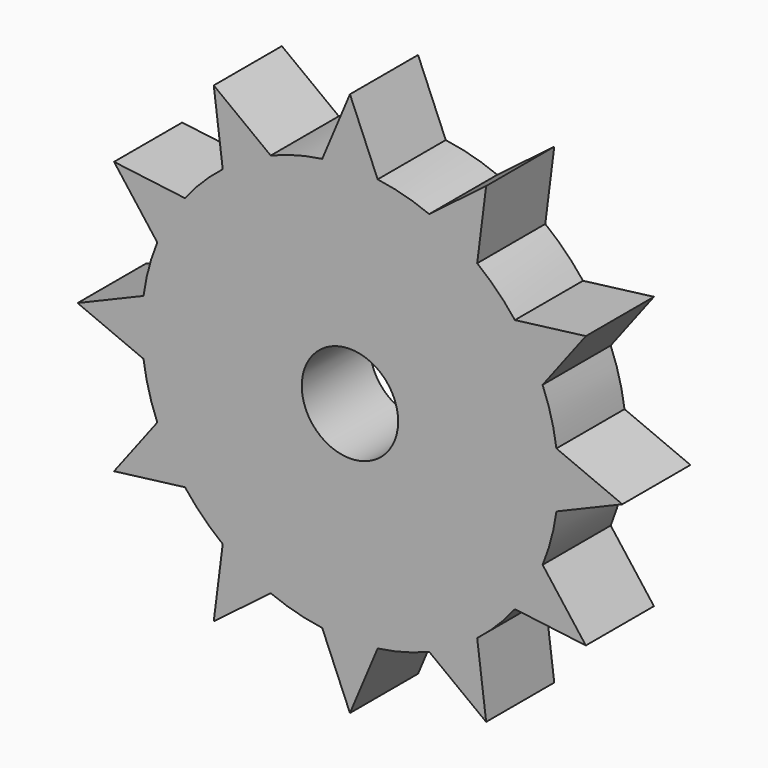
from build123d import *

# Parameters (mm, degrees)
F0_R            = 61.184507213
F1_DEPTH        = 25
F2_R            = 14.1604507034
F3_DEPTH        = 25
F5_DEPTH        = 25
F5_COPIES_COUNT = 12


# Not quite as in the source:
# - a pattern or mirror of a feature is missing from the dataset's text; its kind, count and spacing are read off the source's solid


with BuildPart() as f1:
    # F0 (on Front) → F1 (new body)
    with BuildSketch(Plane.XZ):
        Circle(F0_R)
    extrude(amount=F1_DEPTH)

    # F2 (on face) → F3 (cut)
    with BuildSketch(Plane.XZ.offset(25)):
        Circle(F2_R)
    extrude(amount=-F3_DEPTH, mode=Mode.SUBTRACT)

    # F4 (on Front) → F5 (join)
    with BuildSketch(Plane.XZ):
        with BuildLine():
            Line((0, 80), (-8.1378884566, 60.6408995181))
            ThreePointArc((-8.1378884566, 60.6408995181), (0, 61.184507213), (8.1378884566, 60.6408995181))
            Line((8.1378884566, 60.6408995181), (0, 80))
        make_face()
    f5 = extrude(amount=F5_DEPTH)

    # F5_copies: F5 ×12 about axis
    f5_copies_axis = Axis((0, 0, 0), (0, 1, 0))
    for i in range(1, F5_COPIES_COUNT):
        add(f5.rotate(f5_copies_axis, i * 360 / F5_COPIES_COUNT))


solid = f1.part
